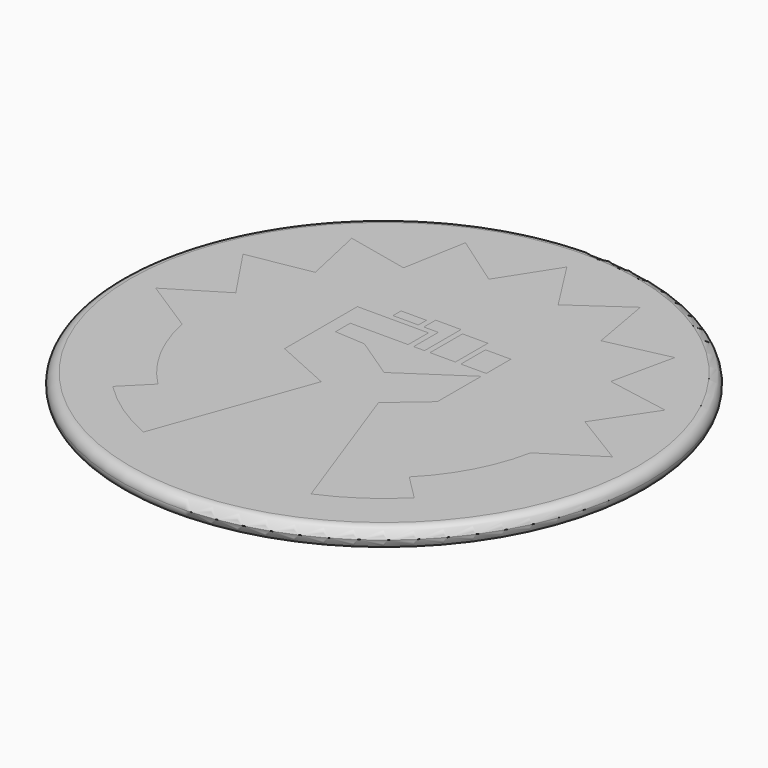
from build123d import *

# Parameters (mm, degrees)
F0_R     = 33.02
F1_DEPTH = 1.27
F0_W     = 3.175
F0_H     = 3.8530217187
F0_H_2   = 5.08
F0_H_3   = 1.27
F2_DEPTH = 1.27
F3_DEPTH = 1.27
F4_R     = 1.26999


# Not quite as in the source:
# - a fillet or chamfer is up to 0.001 mm smaller than in the source, because OpenCascade refuses the exact size


with BuildPart() as f1:
    # F0 (on Top) → F1 (new body)
    with BuildSketch(Plane.XY):
        Circle(F0_R)
        with BuildLine():
            Line((-2.9765482984, 6.0750994888), (-1.8481521045, 6.0750994888))
            Line((-1.8481521045, 6.0750994888), (-1.8481521045, 9.2500994888))
            Line((-1.8481521045, 9.2500994888), (-10.7381521045, 9.2500994888))
            Line((-10.7381521045, 9.2500994888), (-10.7381521045, 2.1359512564))
            Line((-10.7381521045, 2.1359512564), (-10.7381521045, 0))
            Line((-10.7381521045, 0), (-10.7381521045, -2.1359512564))
            Line((-10.7381521045, -2.1359512564), (-3.5774542134, -5.3540385915))
            Line((-3.5774542134, -5.3540385915), (-10.4815781743, -24.5239764104))
            ThreePointArc((-10.4815781743, -24.5239764104), (-14.9410475085, -22.0919442184), (-18.8585378542, -18.8585378542))
            Line((-18.8585378542, -18.8585378542), (-15.7154482119, -15.7154482119))
            ThreePointArc((-15.7154482119, -15.7154482119), (-19.6007001001, -10.476792476), (-21.797952857, -4.3358824068))
            Line((-21.797952857, -4.3358824068), (-28.575, 0))
            Line((-28.575, 0), (-21.8411747772, 4.1126280349))
            Line((-21.8411747772, 4.1126280349), (-26.3998576415, 10.9351790798))
            Line((-26.3998576415, 10.9351790798), (-18.4794121334, 12.3475484289))
            Line((-18.4794121334, 12.3475484289), (-20.2055762724, 20.2055762724))
            Line((-20.2055762724, 20.2055762724), (-12.3475484289, 18.4794121334))
            Line((-12.3475484289, 18.4794121334), (-10.9351790798, 26.3998576415))
            Line((-10.9351790798, 26.3998576415), (-4.3358824068, 21.797952857))
            Line((-4.3358824068, 21.797952857), (0, 28.575))
            Line((0, 28.575), (4.3358824068, 21.797952857))
            Line((4.3358824068, 21.797952857), (10.9351790798, 26.3998576415))
            Line((10.9351790798, 26.3998576415), (12.3475484289, 18.4794121334))
            Line((12.3475484289, 18.4794121334), (20.2055762724, 20.2055762724))
            Line((20.2055762724, 20.2055762724), (18.4794121334, 12.3475484289))
            Line((18.4794121334, 12.3475484289), (26.3998576415, 10.9351790798))
            Line((26.3998576415, 10.9351790798), (21.8411747772, 4.1126280349))
            Line((21.8411747772, 4.1126280349), (28.575, 0))
            Line((28.575, 0), (21.797952857, -4.3358824068))
            ThreePointArc((21.797952857, -4.3358824068), (19.6007001001, -10.476792476), (15.7154482119, -15.7154482119))
            Line((15.7154482119, -15.7154482119), (18.8585378542, -18.8585378542))
            ThreePointArc((18.8585378542, -18.8585378542), (14.9400123163, -22.092644296), (10.4792798584, -24.5249585861))
            Line((10.4792798584, -24.5249585861), (3.5532282388, -5.3177818583))
            Line((3.5532282388, -5.3177818583), (7.9197480572, -1.5753358351))
            Line((7.9197480572, -1.5753358351), (7.9197480572, 0))
            Line((7.9197480572, 0), (7.9197480572, 1.5753358351))
            Line((7.9197480572, 1.5753358351), (7.9197480572, 5.2918064695))
            Line((7.9197480572, 5.2918064695), (5.2798320381, 3.5278709797))
            Line((5.2798320381, 3.5278709797), (0, 0))
            Line((0, 0), (-5.2798320381, 3.5278709797))
            Line((-5.2798320381, 3.5278709797), (-9.0920289037, 3.7660416814))
            Line((-9.0920289037, 3.7660416814), (-9.0920289037, 6.0750994888))
            Line((-9.0920289037, 6.0750994888), (-3.6623482984, 6.0750994888))
            Line((-3.6623482984, 6.0750994888), (-2.9765482984, 6.0750994888))
        make_face(mode=Mode.SUBTRACT)
    extrude(amount=F1_DEPTH)



with BuildPart() as f1b:
    # F0 (on Top) → F1, piece 2 (new body)
    with BuildSketch(Plane.XY):
        with Locations((6.3322480572, 8.0016103481)):
            Rectangle(F0_W, F0_H)
    extrude(amount=F1_DEPTH)


with BuildPart() as f1c:
    # F0 (on Top) → F1, piece 3 (new body)
    with BuildSketch(Plane.XY):
        with Locations((2.4717517016, 8.6150994888)):
            Rectangle(F0_W, F0_H_2)
    extrude(amount=F1_DEPTH)


with BuildPart() as f1d:
    # F0 (on Top) → F1, piece 4 (new body)
    with BuildSketch(Plane.XY):
        Polygon((-1.1623521045, 6.0750994888), (0.1984517016, 6.0750994888), (0.1984517016, 11.7900994888), (-2.9765482984, 11.7900994888), (-2.9765482984, 9.9358994888), (-1.1623521045, 9.9358994888), align=None)
    extrude(amount=F1_DEPTH)


with BuildPart() as f1e:
    # F0 (on Top) → F1, piece 5 (new body)
    with BuildSketch(Plane.XY):
        with Locations((-5.2498482984, 10.5708994888)):
            Rectangle(F0_W, F0_H_3)
    extrude(amount=F1_DEPTH)


with BuildPart() as f2:
    # F0 (on Top) → F2 (new body)
    with BuildSketch(Plane.XY):
        with BuildLine():
            Line((-1.8481521045, 9.2500994888), (-1.8481521045, 6.0750994888))
            Line((-1.8481521045, 6.0750994888), (-2.9765482984, 6.0750994888))
            Line((-2.9765482984, 6.0750994888), (-3.6623482984, 6.0750994888))
            Line((-3.6623482984, 6.0750994888), (-9.0920289037, 6.0750994888))
            Line((-9.0920289037, 6.0750994888), (-9.0920289037, 3.7660416814))
            Line((-9.0920289037, 3.7660416814), (-5.2798320381, 3.5278709797))
            Line((-5.2798320381, 3.5278709797), (0, 0))
            Line((0, 0), (5.2798320381, 3.5278709797))
            Line((5.2798320381, 3.5278709797), (7.9197480572, 5.2918064695))
            Line((7.9197480572, 5.2918064695), (7.9197480572, 1.5753358351))
            Line((7.9197480572, 1.5753358351), (7.9197480572, 0))
            Line((7.9197480572, 0), (7.9197480572, -1.5753358351))
            Line((7.9197480572, -1.5753358351), (3.5532282388, -5.3177818583))
            Line((3.5532282388, -5.3177818583), (10.4792798584, -24.5249585861))
            ThreePointArc((10.4792798584, -24.5249585861), (14.9400123163, -22.092644296), (18.8585378542, -18.8585378542))
            Line((18.8585378542, -18.8585378542), (15.7154482119, -15.7154482119))
            ThreePointArc((15.7154482119, -15.7154482119), (19.6007001001, -10.476792476), (21.797952857, -4.3358824068))
            Line((21.797952857, -4.3358824068), (28.575, 0))
            Line((28.575, 0), (21.8411747772, 4.1126280349))
            Line((21.8411747772, 4.1126280349), (26.3998576415, 10.9351790798))
            Line((26.3998576415, 10.9351790798), (18.4794121334, 12.3475484289))
            Line((18.4794121334, 12.3475484289), (20.2055762724, 20.2055762724))
            Line((20.2055762724, 20.2055762724), (12.3475484289, 18.4794121334))
            Line((12.3475484289, 18.4794121334), (10.9351790798, 26.3998576415))
            Line((10.9351790798, 26.3998576415), (4.3358824068, 21.797952857))
            Line((4.3358824068, 21.797952857), (0, 28.575))
            Line((0, 28.575), (-4.3358824068, 21.797952857))
            Line((-4.3358824068, 21.797952857), (-10.9351790798, 26.3998576415))
            Line((-10.9351790798, 26.3998576415), (-12.3475484289, 18.4794121334))
            Line((-12.3475484289, 18.4794121334), (-20.2055762724, 20.2055762724))
            Line((-20.2055762724, 20.2055762724), (-18.4794121334, 12.3475484289))
            Line((-18.4794121334, 12.3475484289), (-26.3998576415, 10.9351790798))
            Line((-26.3998576415, 10.9351790798), (-21.8411747772, 4.1126280349))
            Line((-21.8411747772, 4.1126280349), (-28.575, 0))
            Line((-28.575, 0), (-21.797952857, -4.3358824068))
            ThreePointArc((-21.797952857, -4.3358824068), (-19.6007001001, -10.476792476), (-15.7154482119, -15.7154482119))
            Line((-15.7154482119, -15.7154482119), (-18.8585378542, -18.8585378542))
            ThreePointArc((-18.8585378542, -18.8585378542), (-14.9410475085, -22.0919442184), (-10.4815781743, -24.5239764104))
            Line((-10.4815781743, -24.5239764104), (-3.5774542134, -5.3540385915))
            Line((-3.5774542134, -5.3540385915), (-10.7381521045, -2.1359512564))
            Line((-10.7381521045, -2.1359512564), (-10.7381521045, 0))
            Line((-10.7381521045, 0), (-10.7381521045, 2.1359512564))
            Line((-10.7381521045, 2.1359512564), (-10.7381521045, 9.2500994888))
            Line((-10.7381521045, 9.2500994888), (-1.8481521045, 9.2500994888))
        make_face()
        with Locations((-5.2498482984, 10.5708994888)):
            Rectangle(F0_W, F0_H_3, mode=Mode.SUBTRACT)
        Polygon((0.1984517016, 11.7900994888), (0.1984517016, 6.0750994888), (-1.1623521045, 6.0750994888), (-1.1623521045, 9.9358994888), (-2.9765482984, 9.9358994888), (-2.9765482984, 11.7900994888), align=None, mode=Mode.SUBTRACT)
        with Locations((6.3322480572, 8.0016103481)):
            Rectangle(F0_W, F0_H, mode=Mode.SUBTRACT)
        with Locations((2.4717517016, 8.6150994888)):
            Rectangle(F0_W, F0_H_2, mode=Mode.SUBTRACT)
    extrude(amount=F2_DEPTH)


with BuildPart() as f1_1:
    add(f1.part)

    add(f1b.part)  # F3 merges F1b

    add(f1c.part)  # F3 merges F1c

    add(f1d.part)  # F3 merges F1d

    add(f1e.part)  # F3 merges F1e
    # F0 (on Top) → F3 (join)
    with BuildSketch(Plane.XY):
        Circle(F0_R)
        with BuildLine():
            Line((-2.9765482984, 6.0750994888), (-1.8481521045, 6.0750994888))
            Line((-1.8481521045, 6.0750994888), (-1.8481521045, 9.2500994888))
            Line((-1.8481521045, 9.2500994888), (-10.7381521045, 9.2500994888))
            Line((-10.7381521045, 9.2500994888), (-10.7381521045, 2.1359512564))
            Line((-10.7381521045, 2.1359512564), (-10.7381521045, 0))
            Line((-10.7381521045, 0), (-10.7381521045, -2.1359512564))
            Line((-10.7381521045, -2.1359512564), (-3.5774542134, -5.3540385915))
            Line((-3.5774542134, -5.3540385915), (-10.4815781743, -24.5239764104))
            ThreePointArc((-10.4815781743, -24.5239764104), (-14.9410475085, -22.0919442184), (-18.8585378542, -18.8585378542))
            Line((-18.8585378542, -18.8585378542), (-15.7154482119, -15.7154482119))
            ThreePointArc((-15.7154482119, -15.7154482119), (-19.6007001001, -10.476792476), (-21.797952857, -4.3358824068))
            Line((-21.797952857, -4.3358824068), (-28.575, 0))
            Line((-28.575, 0), (-21.8411747772, 4.1126280349))
            Line((-21.8411747772, 4.1126280349), (-26.3998576415, 10.9351790798))
            Line((-26.3998576415, 10.9351790798), (-18.4794121334, 12.3475484289))
            Line((-18.4794121334, 12.3475484289), (-20.2055762724, 20.2055762724))
            Line((-20.2055762724, 20.2055762724), (-12.3475484289, 18.4794121334))
            Line((-12.3475484289, 18.4794121334), (-10.9351790798, 26.3998576415))
            Line((-10.9351790798, 26.3998576415), (-4.3358824068, 21.797952857))
            Line((-4.3358824068, 21.797952857), (0, 28.575))
            Line((0, 28.575), (4.3358824068, 21.797952857))
            Line((4.3358824068, 21.797952857), (10.9351790798, 26.3998576415))
            Line((10.9351790798, 26.3998576415), (12.3475484289, 18.4794121334))
            Line((12.3475484289, 18.4794121334), (20.2055762724, 20.2055762724))
            Line((20.2055762724, 20.2055762724), (18.4794121334, 12.3475484289))
            Line((18.4794121334, 12.3475484289), (26.3998576415, 10.9351790798))
            Line((26.3998576415, 10.9351790798), (21.8411747772, 4.1126280349))
            Line((21.8411747772, 4.1126280349), (28.575, 0))
            Line((28.575, 0), (21.797952857, -4.3358824068))
            ThreePointArc((21.797952857, -4.3358824068), (19.6007001001, -10.476792476), (15.7154482119, -15.7154482119))
            Line((15.7154482119, -15.7154482119), (18.8585378542, -18.8585378542))
            ThreePointArc((18.8585378542, -18.8585378542), (14.9400123163, -22.092644296), (10.4792798584, -24.5249585861))
            Line((10.4792798584, -24.5249585861), (3.5532282388, -5.3177818583))
            Line((3.5532282388, -5.3177818583), (7.9197480572, -1.5753358351))
            Line((7.9197480572, -1.5753358351), (7.9197480572, 0))
            Line((7.9197480572, 0), (7.9197480572, 1.5753358351))
            Line((7.9197480572, 1.5753358351), (7.9197480572, 5.2918064695))
            Line((7.9197480572, 5.2918064695), (5.2798320381, 3.5278709797))
            Line((5.2798320381, 3.5278709797), (0, 0))
            Line((0, 0), (-5.2798320381, 3.5278709797))
            Line((-5.2798320381, 3.5278709797), (-9.0920289037, 3.7660416814))
            Line((-9.0920289037, 3.7660416814), (-9.0920289037, 6.0750994888))
            Line((-9.0920289037, 6.0750994888), (-3.6623482984, 6.0750994888))
            Line((-3.6623482984, 6.0750994888), (-2.9765482984, 6.0750994888))
        make_face(mode=Mode.SUBTRACT)
        with BuildLine():
            Line((-1.8481521045, 9.2500994888), (-1.8481521045, 6.0750994888))
            Line((-1.8481521045, 6.0750994888), (-2.9765482984, 6.0750994888))
            Line((-2.9765482984, 6.0750994888), (-3.6623482984, 6.0750994888))
            Line((-3.6623482984, 6.0750994888), (-9.0920289037, 6.0750994888))
            Line((-9.0920289037, 6.0750994888), (-9.0920289037, 3.7660416814))
            Line((-9.0920289037, 3.7660416814), (-5.2798320381, 3.5278709797))
            Line((-5.2798320381, 3.5278709797), (0, 0))
            Line((0, 0), (5.2798320381, 3.5278709797))
            Line((5.2798320381, 3.5278709797), (7.9197480572, 5.2918064695))
            Line((7.9197480572, 5.2918064695), (7.9197480572, 1.5753358351))
            Line((7.9197480572, 1.5753358351), (7.9197480572, 0))
            Line((7.9197480572, 0), (7.9197480572, -1.5753358351))
            Line((7.9197480572, -1.5753358351), (3.5532282388, -5.3177818583))
            Line((3.5532282388, -5.3177818583), (10.4792798584, -24.5249585861))
            ThreePointArc((10.4792798584, -24.5249585861), (14.9400123163, -22.092644296), (18.8585378542, -18.8585378542))
            Line((18.8585378542, -18.8585378542), (15.7154482119, -15.7154482119))
            ThreePointArc((15.7154482119, -15.7154482119), (19.6007001001, -10.476792476), (21.797952857, -4.3358824068))
            Line((21.797952857, -4.3358824068), (28.575, 0))
            Line((28.575, 0), (21.8411747772, 4.1126280349))
            Line((21.8411747772, 4.1126280349), (26.3998576415, 10.9351790798))
            Line((26.3998576415, 10.9351790798), (18.4794121334, 12.3475484289))
            Line((18.4794121334, 12.3475484289), (20.2055762724, 20.2055762724))
            Line((20.2055762724, 20.2055762724), (12.3475484289, 18.4794121334))
            Line((12.3475484289, 18.4794121334), (10.9351790798, 26.3998576415))
            Line((10.9351790798, 26.3998576415), (4.3358824068, 21.797952857))
            Line((4.3358824068, 21.797952857), (0, 28.575))
            Line((0, 28.575), (-4.3358824068, 21.797952857))
            Line((-4.3358824068, 21.797952857), (-10.9351790798, 26.3998576415))
            Line((-10.9351790798, 26.3998576415), (-12.3475484289, 18.4794121334))
            Line((-12.3475484289, 18.4794121334), (-20.2055762724, 20.2055762724))
            Line((-20.2055762724, 20.2055762724), (-18.4794121334, 12.3475484289))
            Line((-18.4794121334, 12.3475484289), (-26.3998576415, 10.9351790798))
            Line((-26.3998576415, 10.9351790798), (-21.8411747772, 4.1126280349))
            Line((-21.8411747772, 4.1126280349), (-28.575, 0))
            Line((-28.575, 0), (-21.797952857, -4.3358824068))
            ThreePointArc((-21.797952857, -4.3358824068), (-19.6007001001, -10.476792476), (-15.7154482119, -15.7154482119))
            Line((-15.7154482119, -15.7154482119), (-18.8585378542, -18.8585378542))
            ThreePointArc((-18.8585378542, -18.8585378542), (-14.9410475085, -22.0919442184), (-10.4815781743, -24.5239764104))
            Line((-10.4815781743, -24.5239764104), (-3.5774542134, -5.3540385915))
            Line((-3.5774542134, -5.3540385915), (-10.7381521045, -2.1359512564))
            Line((-10.7381521045, -2.1359512564), (-10.7381521045, 0))
            Line((-10.7381521045, 0), (-10.7381521045, 2.1359512564))
            Line((-10.7381521045, 2.1359512564), (-10.7381521045, 9.2500994888))
            Line((-10.7381521045, 9.2500994888), (-1.8481521045, 9.2500994888))
        make_face()
        with Locations((-5.2498482984, 10.5708994888)):
            Rectangle(F0_W, F0_H_3, mode=Mode.SUBTRACT)
        Polygon((0.1984517016, 11.7900994888), (0.1984517016, 6.0750994888), (-1.1623521045, 6.0750994888), (-1.1623521045, 9.9358994888), (-2.9765482984, 9.9358994888), (-2.9765482984, 11.7900994888), align=None, mode=Mode.SUBTRACT)
        with Locations((6.3322480572, 8.0016103481)):
            Rectangle(F0_W, F0_H, mode=Mode.SUBTRACT)
        with Locations((2.4717517016, 8.6150994888)):
            Rectangle(F0_W, F0_H_2, mode=Mode.SUBTRACT)
        with Locations((6.3322480572, 8.0016103481)):
            Rectangle(F0_W, F0_H)
        with Locations((2.4717517016, 8.6150994888)):
            Rectangle(F0_W, F0_H_2)
        Polygon((-1.1623521045, 6.0750994888), (0.1984517016, 6.0750994888), (0.1984517016, 11.7900994888), (-2.9765482984, 11.7900994888), (-2.9765482984, 9.9358994888), (-1.1623521045, 9.9358994888), align=None)
        with Locations((-5.2498482984, 10.5708994888)):
            Rectangle(F0_W, F0_H_3)
    extrude(amount=-F3_DEPTH)

    # F4 (radius 1.27 in the source; OpenCascade refuses exactly that, so slightly less here)
    f4_edges = [f1_1.edges().sort_by_distance(p)[0] for p in [
        (33.02, 0, 0.635),
        (-33.02, 0, 0),
        (-33.02, 0, 1.27),
        (-33.02, 0, -1.27),
    ]]
    fillet(f4_edges, radius=F4_R)


solid = Compound([f2.part, f1_1.part])
